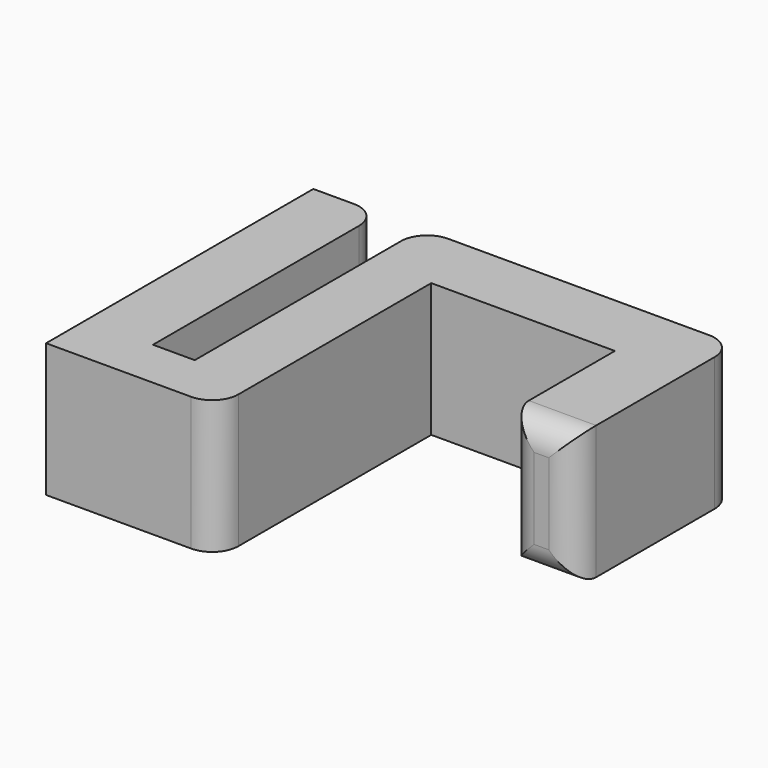
from build123d import *

# Parameters (mm, degrees)
F1_DEPTH     = 25.4
F2_TEXT_SIZE = 19.7831024582
F3_DEPTH     = 2
F4_R         = 5


# Not quite as in the source:
# - Text() gives the source's letters only with a copy of the font that has no kerning and outlines rounded to 1/6400 em; it was checked with that copy


with BuildPart() as f1:
    # F0 (on Top) → F1 (new body)
    with BuildSketch(Plane.XY):
        Polygon((0, 63.5), (0, 0), (32.5752518936, 0), (32.5752518936, 50.8), (67.4797778515, 50.8), (67.4797778515, 25.3516854542), (80.2734648196, 25.3516854542), (80.2734648196, 63.5), (20.6375, 63.5), (20.6375, 9.52754), (12.7, 9.52754), (12.7, 63.5), align=None)
    extrude(amount=F1_DEPTH)

    # F2 (on face) → F3 (cut)
    with BuildSketch(Plane(origin=(0, 0, 0), x_dir=(0, -1, 0), z_dir=(-1, 0, 0))):
        with Locations((-63.5, 6.811771027)):
            Text('Bigbee', F2_TEXT_SIZE, font='Open Sans', text_align=(TextAlign.LEFT, TextAlign.BOTTOM))
    extrude(amount=-F3_DEPTH, mode=Mode.SUBTRACT)

    # F4
    f4_edges = [f1.edges().sort_by_distance(p)[0] for p in [
        (73.876621, 25.351685, 25.4),
        (73.876621, 25.351685, 0),
        (80.273465, 25.351685, 12.7),
        (67.479778, 25.351685, 12.7),
        (80.273465, 63.5, 12.7),
        (32.575252, 0, 12.7),
        (20.6375, 63.5, 12.7),
        (12.7, 63.5, 12.7),
    ]]
    fillet(f4_edges, radius=F4_R)


solid = f1.part
